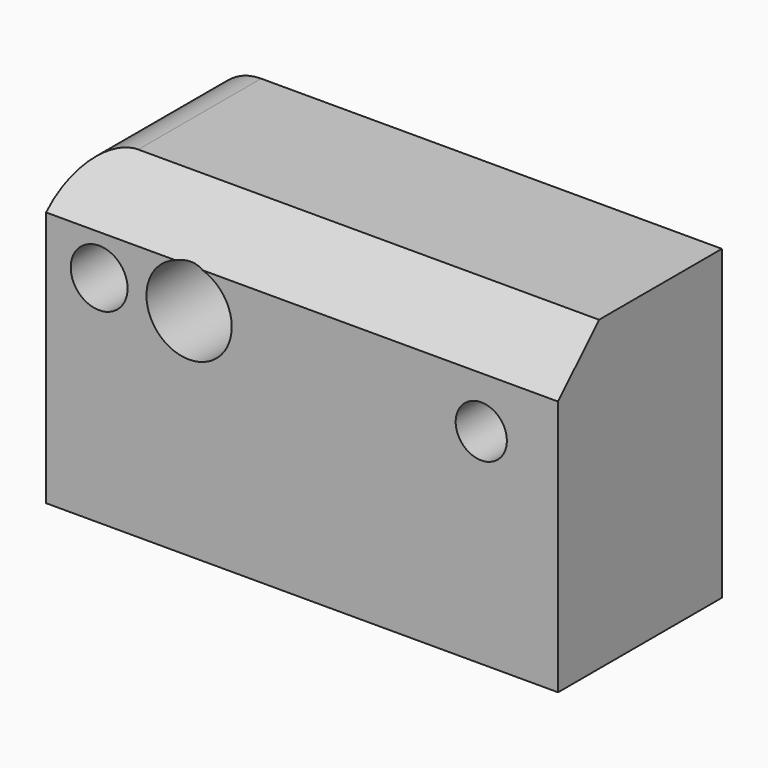
from build123d import *

# Parameters (mm, degrees)
F0_W        = 127
F0_H        = 76.2
F0_R        = 7.0531122836
F0_R_2      = 6.35
F1_DEPTH    = 50.8
F2_R        = 10.5798439837
F3_DEPTH    = 86.868
F4_T1_DEPTH = 192.3207478943
F5_R        = 12.7


# Not quite as in the source:
# - a fillet or chamfer that OpenCascade refuses, or shapes differently, is made with other operations: its cross-section is extruded or revolved along the edge and cut away or added


with BuildPart() as f1:
    # F0 (on Front) → F1 (new body)
    with BuildSketch(Plane.XZ):
        with Locations((0.679500401, -0.9445134997)):
            Rectangle(F0_W, F0_H)
        with Locations((-49.6532134712, 14.4240399823)):
            Circle(F0_R, mode=Mode.SUBTRACT)
        with Locations((45.129500401, 11.7554865003)):
            Circle(F0_R_2, mode=Mode.SUBTRACT)
    extrude(amount=F1_DEPTH)

    # F2 (on face) → F3 (cut)
    with BuildSketch(Plane.XZ.offset(50.8)):
        with Locations((-27.3451898247, 14.4321834669)):
            Circle(F2_R)
    extrude(amount=-F3_DEPTH, mode=Mode.SUBTRACT)

    # F4: chamfer of 12.7 on 1 edges, made by hand

    # F4_s2 → F4_t1 (cut)
    with BuildSketch(Plane.YZ.offset(-95.4808735461)):
        Polygon((-38.1, 37.1554865003), (-50.8, 24.4554865003), (-50.8, 37.1554865003), align=None)
    extrude(amount=F4_T1_DEPTH, mode=Mode.SUBTRACT)

    # F5
    f5_edges = [f1.edges().sort_by_distance(p)[0] for p in [
        (-62.8205, -19.05, 37.155487),
    ]]
    fillet(f5_edges, radius=F5_R)


solid = f1.part
